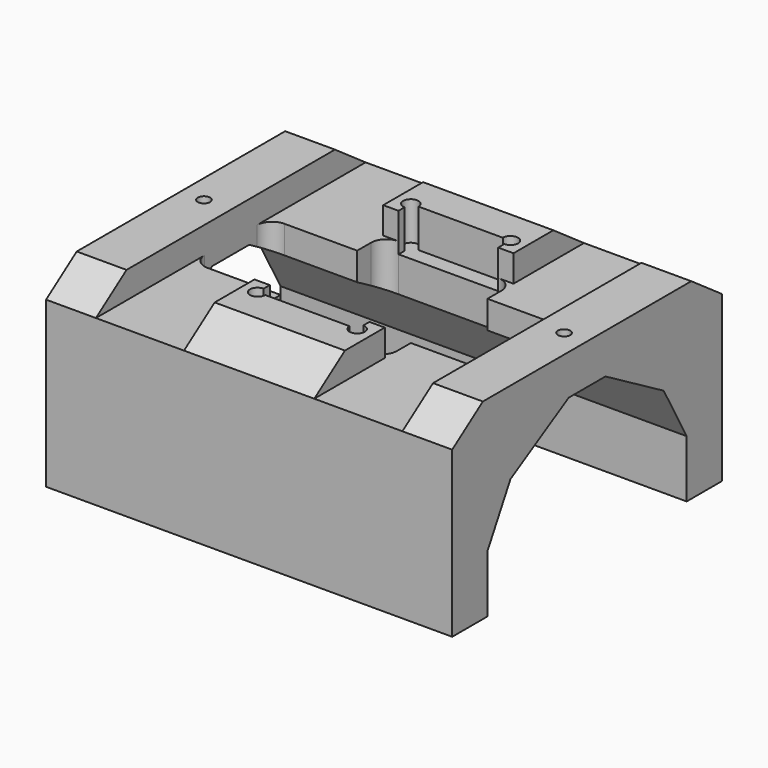
from build123d import *

# Parameters (mm, degrees)
F1_DEPTH  = 53
F2_W      = 80
F2_H      = 25
F3_DEPTH  = 25
F4_W      = 23
F4_H      = 115.9437634051
F5_DEPTH  = 7
F6_W      = 34
F6_H      = 8.5
F7_DEPTH  = 50.001
F8_W      = 26
F8_H      = 4
F9_DEPTH  = 10
F10_R     = 2
F11_DEPTH = 10
F12_SIZE2 = 7
F12_SIZE  = 10
F13_SIZE2 = 10
F13_SIZE  = 7
F15_D     = 3.2
F15_DEPTH = 12
F15_TIP   = 0.9613769904
F16_R     = 3.99999


# Not quite as in the source:
# - a fillet or chamfer is up to 0.001 mm smaller than in the source, because OpenCascade refuses the exact size


with BuildPart() as f1:
    # F0 (on Right) → F1 (new body, symmetric)
    with BuildSketch(Plane.YZ):
        Polygon((44, 25), (-44, 25), (-44, -25), (-32.5, -25), (-32.5, -10), (-25, 3.5), (-6, 14.5), (0, 14.5), (6, 14.5), (25, 3.5), (32.5, -10), (32.5, -25), (44, -25), align=None)
    extrude(amount=F1_DEPTH, both=True)

    # F2 (on face) → F3 (cut)
    with BuildSketch(Plane.XY.offset(25)):
        Rectangle(F2_W, F2_H)
    extrude(amount=-F3_DEPTH, mode=Mode.SUBTRACT)

    # F4 (on face) → F5 (cut)
    with BuildSketch(Plane.XY.offset(25)):
        with Locations((-28.5, -2.7361307293)):
            Rectangle(F4_W, F4_H)
        with Locations((28.5, -2.7361307293)):
            Rectangle(F4_W, F4_H)
    extrude(amount=-F5_DEPTH, mode=Mode.SUBTRACT)

    # F6 (on face) → F7 (cut, through all)
    with BuildSketch(Plane.XY.offset(25)):
        with Locations((0, 16.75)):
            Rectangle(F6_W, F6_H)
        with Locations((0, -16.75)):
            Rectangle(F6_W, F6_H)
    extrude(amount=-F7_DEPTH, mode=Mode.SUBTRACT)

    # F8 (on face) → F9 (cut)
    with BuildSketch(Plane.XY.offset(25)):
        with Locations((0, 23)):
            Rectangle(F8_W, F8_H)
        with Locations((0, -23)):
            Rectangle(F8_W, F8_H)
    extrude(amount=-F9_DEPTH, mode=Mode.SUBTRACT)

    # F10 (on face) → F11 (cut)
    with BuildSketch(Plane.XY.offset(25)):
        with Locations((-13, 25)):
            Circle(F10_R)
        with Locations((13, 25)):
            Circle(F10_R)
        with Locations((-13, -25)):
            Circle(F10_R)
        with Locations((13, -25)):
            Circle(F10_R)
    extrude(amount=-F11_DEPTH, mode=Mode.SUBTRACT)

    # F12
    f12_edges = [f1.edges().sort_by_distance(p)[0] for p in [
        (-46.5, -44, 25),
        (0, -44, 25),
        (46.5, -44, 25),
    ]]
    chamfer(f12_edges, length=F12_SIZE, length2=F12_SIZE2)

    # F13
    f13_edges = [f1.edges().sort_by_distance(p)[0] for p in [
        (-46.5, 44, 25),
        (0, 44, 25),
        (46.5, 44, 25),
    ]]
    f13_side = f1.faces().sort_by_distance((0, 44, -1.390719))[0]
    chamfer(f13_edges, length=F13_SIZE, length2=F13_SIZE2, reference=f13_side)

    # F15
    with Locations(Plane.XY.offset(25)):
        with Locations((-47, 0), (47, 0)):
            Hole(F15_D / 2, depth=F15_DEPTH)
            with Locations((0, 0, -(F15_DEPTH + F15_TIP / 2))):  # 118° drill point
                Cone(0, F15_D / 2, F15_TIP, mode=Mode.SUBTRACT)

    # F16 (radius 4 in the source; OpenCascade refuses exactly that, so slightly less here)
    f16_edges = [f1.edges().sort_by_distance(p)[0] for p in [
        (17, 21, 11.907895),
        (-17, 21, 11.907895),
        (-40, 12.5, 14.368421),
        (-40, -12.5, 14.368421),
        (-17, -21, 11.907895),
        (17, -21, 11.907895),
        (40, -12.5, 14.368421),
        (40, 12.5, 14.368421),
    ]]
    fillet(f16_edges, radius=F16_R)


solid = f1.part
